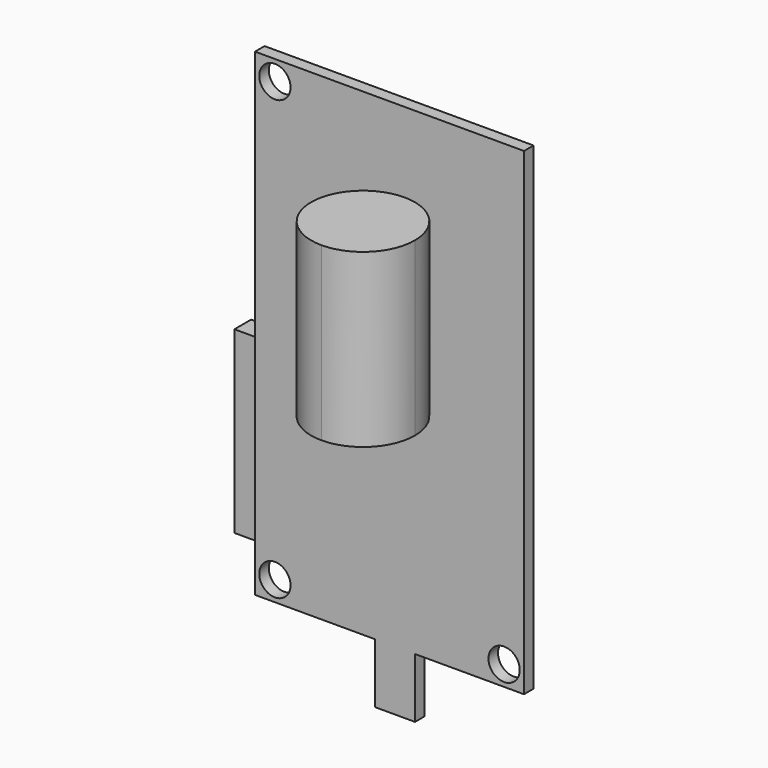
from build123d import *

# Parameters (mm, degrees)
F0_W     = 5.08
F0_H     = 7.62
F1_DEPTH = 1.524
F2_W     = 14
F2_H     = 22.86
F3_DEPTH = 2.66
F6_DEPTH = 21.8948
F7_R     = 1.9939
F8_DEPTH = 14.733


with BuildPart() as f1:
    # F0 (on Front) → F1 (new body)
    with BuildSketch(Plane.XZ):
        Polygon((16.6127808136, 35.4363795967), (-17.6772191864, 35.4363795967), (-17.6772191864, -25.5236204033), (-2.3591062054, -25.5236204033), (2.7208937946, -25.5236204033), (16.6127808136, -25.5236204033), align=None)
        with Locations((0.1808937946, -29.3336204033)):
            Rectangle(F0_W, F0_H)
    extrude(amount=F1_DEPTH)

    # F2 (on face) → F3 (join)
    with BuildSketch(Plane(origin=(0, 0, 0), x_dir=(-1, 0, 0), z_dir=(0, 1, 0))):
        with Locations((14.5172191864, -9.0136204033)):
            Rectangle(F2_W, F2_H)
    extrude(amount=F3_DEPTH)

    # F7 (on face) → F8 (cut, through all)
    with BuildSketch(Plane(origin=(0, 0, 0), x_dir=(-1, 0, 0), z_dir=(0, 1, 0))):
        with Locations((15.1372191864, 32.8963795967)):
            Circle(F7_R)
        with Locations((15.1372191864, -22.9836204033)):
            Circle(F7_R)
        with Locations((-14.0727808136, -22.9836204033)):
            Circle(F7_R)
    extrude(amount=-F8_DEPTH, mode=Mode.SUBTRACT)


with BuildPart() as f6:
    # F5 (on offset) → F6 (new body)
    with BuildSketch(Plane.XY.offset(25.2763795967)):
        with BuildLine():
            ThreePointArc((7.9767808136, -8.128), (6.0425139965, -3.458266817), (1.3727808136, -1.524))
            Line((1.3727808136, -1.524), (1.3727808136, -14.732))
            ThreePointArc((1.3727808136, -14.732), (6.0425139965, -12.797733183), (7.9767808136, -8.128))
        make_face()
        with BuildLine():
            Line((1.3727808136, -14.732), (1.3727808136, -1.524))
            ThreePointArc((1.3727808136, -1.524), (-5.2312191864, -8.128), (1.3727808136, -14.732))
        make_face()
    extrude(amount=-F6_DEPTH)


solid = Compound([f1.part, f6.part])
